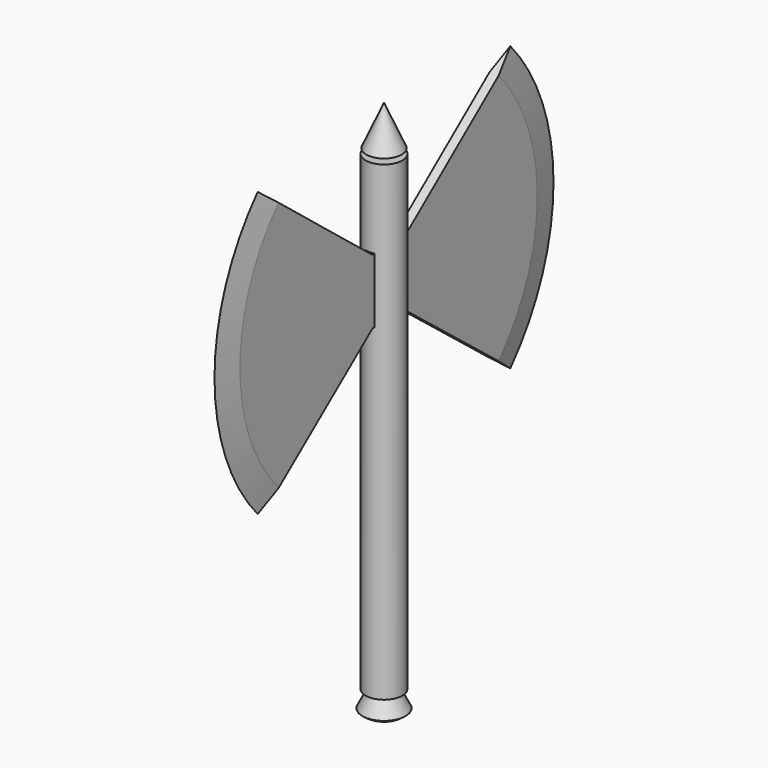
from build123d import *

# Parameters (mm, degrees)
F0_R          = 20
F1_DEPTH      = 324
F1_DEPTH_BACK = 191
F3_DEPTH      = 5
F4_SIZE2      = 28.356399
F4_SIZE       = 4.99999


# Not quite as in the source:
# - a fillet or chamfer is up to 0.001 mm smaller than in the source, because OpenCascade refuses the exact size


with BuildPart() as f1:
    # F0 (on Top) → F1 (new body, two sides)
    with BuildSketch(Plane.XY) as f1_sk:
        Circle(F0_R)
    extrude(amount=F1_DEPTH)
    extrude(f1_sk.sketch, amount=-F1_DEPTH_BACK)

    # F2 (on Right) → F3 (join)
    with BuildSketch(Plane.YZ):
        with BuildLine():
            Line((9.8391985521, 165.7918989658), (21.8501202762, 166.5147198653))
            Line((21.8501202762, 166.5147198653), (172.5762003339, 47.3351646042))
            ThreePointArc((172.5762003339, 47.3351646042), (231.5665738369, 202.382288244), (172.5762003339, 357.4294118838))
            Line((172.5762003339, 357.4294118838), (22.4253297422, 237.5259771443))
            Line((22.4253297422, 237.5259771443), (9.8391985521, 237.5259771443))
            Line((9.8391985521, 237.5259771443), (9.8391985521, 165.7918989658))
        make_face()
    extrude(amount=F3_DEPTH)

    # F4 (size 5 and 28.3564090981 in the source; OpenCascade refuses exactly that, so slightly less here)
    f4_edges = [f1.edges().sort_by_distance(p)[0] for p in [
        (5, 231.566574, 202.382288),
    ]]
    f4_side = f1.faces().sort_by_distance((2.5, 231.566574, 202.382288))[0]
    chamfer(f4_edges, length=F4_SIZE, length2=F4_SIZE2, reference=f4_side)

    # F5: F1 across plane


with BuildPart() as f1_1:
    add(f1.part)
    add(f1.part.mirror(Plane.YZ))

    # F6: F1 across plane


with BuildPart() as f1_2:
    add(f1_1.part)
    add(f1_1.part.mirror(Plane.XZ))

    # F7 (on Right) → F8 (revolve)
    with BuildSketch(Plane.YZ):
        Polygon((5.505359266, 312.6185536385), (5.505359266, 329.4300734997), (19.3500220776, 329.4300734997), (0, 373.1769025326), (0, 329.4300734997), (0, 312.6185536385), align=None)
    revolve(axis=Axis((0, 0, 351.3034880161), (0, 0, -1)))

    # F9 (on Right) → F10 (revolve)
    with BuildSketch(Plane.YZ):
        with BuildLine():
            Line((-15.0489732623, -187.7072155476), (-15.0489732623, -192.4124807119))
            Line((-15.0489732623, -192.4124807119), (-23.5689829473, -209.4524800777))
            ThreePointArc((-23.5689829473, -209.4524800777), (-12.5456612149, -215.444084642), (0, -215.3050452471))
            Line((0, -215.3050452471), (0, -209.4524800777))
            Line((0, -209.4524800777), (0, -193.2779252529))
            Line((0, -193.2779252529), (0, -187.7072155476))
            Line((0, -187.7072155476), (-15.0489732623, -187.7072155476))
        make_face()
    revolve(axis=Axis((0, 0, -201.3652026653), (0, 0, -1)))


solid = f1_2.part
